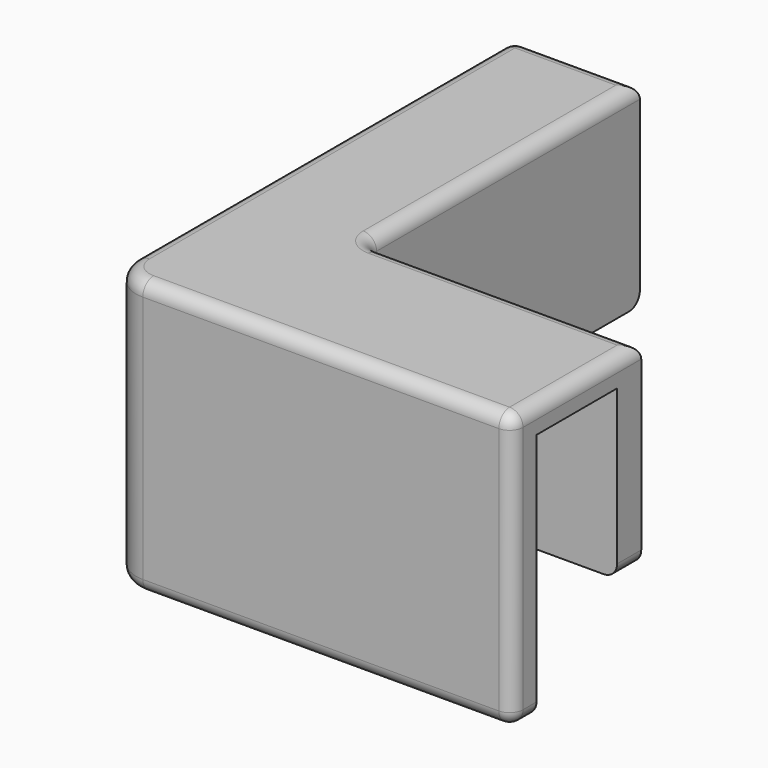
from build123d import *

# Parameters (mm, degrees)
F1_DEPTH    = 4
F3_DEPTH    = 25
F5_DEPTH    = 12
F6_R        = 2
F7_T1_DEPTH = 41
F7_T4_ANGLE = 90
F7_T6_ANGLE = 90


# Not quite as in the source:
# - a fillet or chamfer that OpenCascade refuses, or shapes differently, is made with other operations: its cross-section is extruded or revolved along the edge and cut away or added


with BuildPart() as f1:
    # F0 (on Top) → F1 (new body)
    with BuildSketch(Plane.XY):
        Polygon((7, 12), (7, 63), (-12, 63), (-12, -12), (48, -12), (48, 12), align=None)
    extrude(amount=F1_DEPTH)

    # F2 (on face) → F3 (join)
    with BuildSketch(Plane(origin=(0, 0, 0), x_dir=(1, 0, 0), z_dir=(0, 0, -1))):
        Polygon((48, 12), (-12, 12), (-12, -63), (-7.5, -63), (-7.5, 7.5), (48, 7.5), align=None)
        Polygon((2.5, -63), (7, -63), (7, -12), (48, -12), (48, -7.5), (2.5, -7.5), align=None)
    extrude(amount=F3_DEPTH)

    # F4 (on face) → F5 (join)
    with BuildSketch(Plane(origin=(0, 0, -25), x_dir=(1, 0, 0), z_dir=(0, 0, -1))):
        Polygon((48, 12), (-12, 12), (-12, -63), (-7.5, -63), (-7.5, 7.5), (48, 7.5), align=None)
    extrude(amount=F5_DEPTH)

    # F6
    f6_edges = [f1.edges().sort_by_distance(p)[0] for p in [
        (7, 37.5, 4),
        (-2.5, 63, 4),
        (-12, 25.5, 4),
        (18, -12, 4),
        (48, 0, 4),
        (27.5, 12, 4),
        (-9.75, 63, -37),
        (4.75, 63, -25),
        (48, -9.75, -37),
        (48, 9.75, -25),
        (2.5, 7.5, -12.5),
        (7, 12, -10.5),
        (-12, 63, -16.5),
        (48, -12, -16.5),
        (-12, 25.5, -37),
        (18, -12, -37),
    ]]
    fillet(f6_edges, radius=F6_R)

    # F7: fillet of radius 5 on 1 edges, made by hand

    # F7_s2 → F7_t1 (cut)
    with BuildSketch(Plane.XY.offset(-37)):
        with BuildLine():
            ThreePointArc((-12, -7), (-10.5355339059, -10.5355339059), (-7, -12))
            Line((-7, -12), (-12, -12))
            Line((-12, -12), (-12, -7))
        make_face()
    extrude(amount=F7_T1_DEPTH, mode=Mode.SUBTRACT)

    # F7_s3 → F7_t4 (revolve, cut)
    with BuildSketch(Plane.YZ.offset(-7)):
        with BuildLine():
            ThreePointArc((-10, -37), (-11.4142135624, -36.4142135624), (-12, -35))
            Line((-12, -35), (-12, -37))
            Line((-12, -37), (-10, -37))
        make_face()
    revolve(axis=Axis((-7, -7, -37), (0, 0, -1)), revolution_arc=F7_T4_ANGLE, mode=Mode.SUBTRACT)

    # F7_s5 → F7_t6 (revolve, cut)
    with BuildSketch(Plane.XZ.offset(7)):
        with BuildLine():
            ThreePointArc((-10, 4), (-11.4142135624, 3.4142135624), (-12, 2))
            Line((-12, 2), (-12, 4))
            Line((-12, 4), (-10, 4))
        make_face()
    revolve(axis=Axis((-7, -7, 4), (0, 0, 1)), revolution_arc=F7_T6_ANGLE, mode=Mode.SUBTRACT)


solid = f1.part
